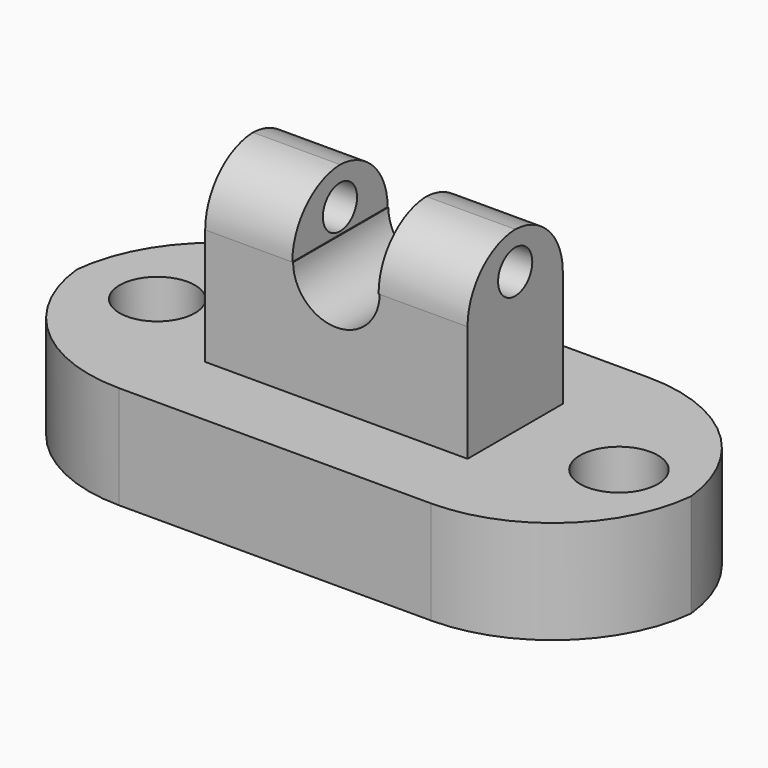
from build123d import *

# Parameters (mm, degrees)
F0_W         = 151.6868472099
F0_H         = 67.0943334699
F1_DEPTH     = 25.4
F9_T1_DEPTH  = 212.7476366747
F2_R         = 9.5743665409
F2_R_2       = 9.2989273841
F3_DEPTH     = 25.401
F4_W         = 64.6063834429
F4_H         = 29.3284505606
F10_DEPTH    = 43.7951106578
F11_T1_DEPTH = 140.443628516
F5_R         = 5.2641428602
F6_DEPTH     = 107.9417508016
F8_DEPTH     = 48.2123920152


# Not quite as in the source:
# - a fillet or chamfer that OpenCascade refuses, or shapes differently, is made with other operations: its cross-section is extruded or revolved along the edge and cut away or added


with BuildPart() as f1:
    # F0 (on Top) → F1 (new body)
    with BuildSketch(Plane.XY):
        Rectangle(F0_W, F0_H)
    extrude(amount=F1_DEPTH)

    # F9: fillet of radius 37.4695273349 on 4 edges, made by hand

    # F9_s2 → F9_t1 (cut)
    with BuildSketch(Plane.XY.offset(-93.6738183373)):
        with BuildLine():
            ThreePointArc((75.843423605, -3.9223606), (64.8688531364, 22.5725962664), (38.37389627, 33.5471667349))
            Line((38.37389627, 33.5471667349), (75.843423605, 33.5471667349))
            Line((75.843423605, 33.5471667349), (75.843423605, -3.9223606))
        make_face()
        with BuildLine():
            ThreePointArc((75.843423605, 3.9223606), (64.8688531364, -22.5725962664), (38.37389627, -33.5471667349))
            Line((38.37389627, -33.5471667349), (75.843423605, -33.5471667349))
            Line((75.843423605, -33.5471667349), (75.843423605, 3.9223606))
        make_face()
        with BuildLine():
            ThreePointArc((-75.843423605, 3.9223606), (-64.8688531364, -22.5725962664), (-38.37389627, -33.5471667349))
            Line((-38.37389627, -33.5471667349), (-75.843423605, -33.5471667349))
            Line((-75.843423605, -33.5471667349), (-75.843423605, 3.9223606))
        make_face()
        with BuildLine():
            ThreePointArc((-38.37389627, 33.5471667349), (-64.8688531364, 22.5725962664), (-75.843423605, -3.9223606))
            Line((-75.843423605, -3.9223606), (-75.843423605, 33.5471667349))
            Line((-75.843423605, 33.5471667349), (-38.37389627, 33.5471667349))
        make_face()
    extrude(amount=F9_T1_DEPTH, mode=Mode.SUBTRACT)

    # F2 (on face) → F3 (cut, through all)
    with BuildSketch(Plane.XY.offset(25.4)):
        with Locations((57.8670687973, 0)):
            Circle(F2_R)
        with Locations((-55.8316037059, 0)):
            Circle(F2_R_2)
    extrude(amount=-F3_DEPTH, mode=Mode.SUBTRACT)

    # F4 (on face) → F10 (join)
    with BuildSketch(Plane.XY.offset(25.4)):
        Rectangle(F4_W, F4_H)
    extrude(amount=F10_DEPTH)

    # F11: fillet of radius 15.1674490146 on 2 edges, made by hand

    # F11_s2 → F11_t1 (cut)
    with BuildSketch(Plane.YZ.offset(-70.221814258)):
        with BuildLine():
            ThreePointArc((-14.6642252803, 54.0276616432), (-10.2217823172, 64.7526676947), (0.5032237343, 69.1951106578))
            Line((0.5032237343, 69.1951106578), (-14.6642252803, 69.1951106578))
            Line((-14.6642252803, 69.1951106578), (-14.6642252803, 54.0276616432))
        make_face()
        with BuildLine():
            ThreePointArc((14.6642252803, 54.0276616432), (10.2217823172, 64.7526676947), (-0.5032237343, 69.1951106578))
            Line((-0.5032237343, 69.1951106578), (14.6642252803, 69.1951106578))
            Line((14.6642252803, 69.1951106578), (14.6642252803, 54.0276616432))
        make_face()
    extrude(amount=F11_T1_DEPTH, mode=Mode.SUBTRACT)

    # F5 (on face) → F6 (cut, through all)
    with BuildSketch(Plane.YZ.offset(32.3031917214)):
        with Locations((0, 59.9929094315)):
            Circle(F5_R)
    extrude(amount=-F6_DEPTH, mode=Mode.SUBTRACT)

    # F7 (on face) → F8 (cut, through all)
    with BuildSketch(Plane.XZ.offset(14.6642252803)):
        with BuildLine():
            Line((-10.8441319317, 74.8410969973), (-10.8441319317, 54.0276616432))
            Line((-10.8441319317, 54.0276616432), (-10.6545253, 54.0276616432))
            ThreePointArc((-10.6545253, 54.0276616432), (-1.1741893399, 64.6172881126), (10.3957206011, 56.3617358819))
            Line((10.3957206011, 56.3617358819), (10.3957206011, 74.8410969973))
            Line((10.3957206011, 74.8410969973), (-10.8441319317, 74.8410969973))
        make_face()
        with BuildLine():
            ThreePointArc((10.3957206011, 56.3617358819), (-1.1741893399, 64.6172881126), (-10.6545253, 54.0276616432))
            Line((-10.6545253, 54.0276616432), (10.3957206011, 54.0276616432))
            Line((10.3957206011, 54.0276616432), (10.3957206011, 56.3617358819))
        make_face()
        with BuildLine():
            Line((10.3957206011, 54.0276616432), (-10.6545253, 54.0276616432))
            ThreePointArc((-10.6545253, 54.0276616432), (0, 43.3731363432), (10.6545253, 54.0276616432))
            Line((10.6545253, 54.0276616432), (10.3957206011, 54.0276616432))
        make_face()
    extrude(amount=-F8_DEPTH, mode=Mode.SUBTRACT)


solid = f1.part
